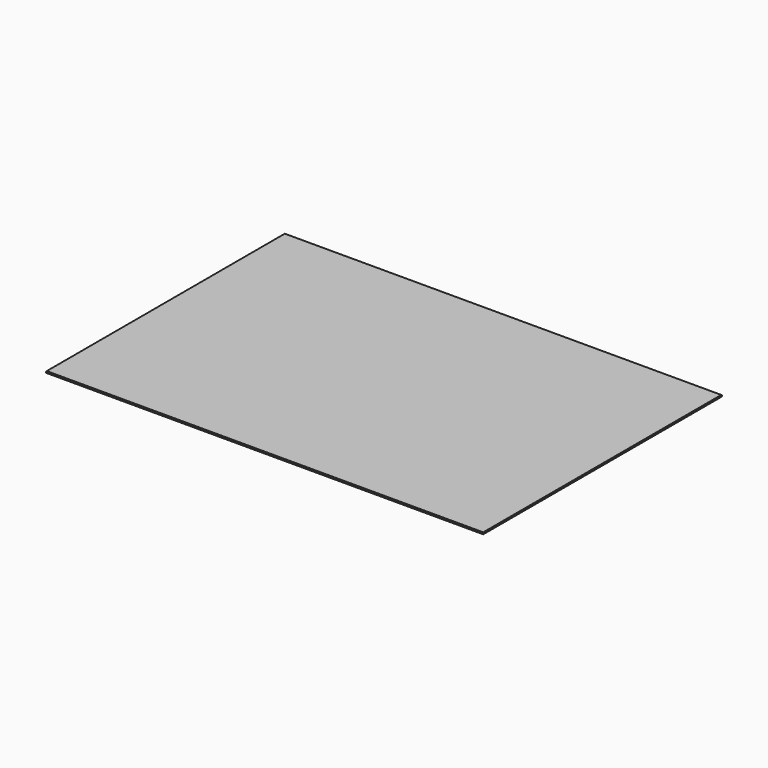
from build123d import *

# Parameters (mm, degrees)
F0_W     = 1221
F0_H     = 833
F1_DEPTH = 2.5
F2_SIZE  = 1
F3_SIZE  = 1


with BuildPart() as f1:
    # F0 (on Top) → F1 (new body, symmetric)
    with BuildSketch(Plane.XY):
        Rectangle(F0_W, F0_H)
    extrude(amount=F1_DEPTH, both=True)

    # F2
    f2_edges = [f1.edges().sort_by_distance(p)[0] for p in [
        (0, -416.5, 2.5),
        (610.5, 0, 2.5),
        (0, 416.5, 2.5),
        (-610.5, 0, 2.5),
    ]]
    chamfer(f2_edges, length=F2_SIZE)

    # F3
    f3_edges = [f1.edges().sort_by_distance(p)[0] for p in [
        (0, 416.5, -2.5),
        (610.5, 0, -2.5),
        (0, -416.5, -2.5),
        (-610.5, 0, -2.5),
    ]]
    chamfer(f3_edges, length=F3_SIZE)


solid = f1.part
